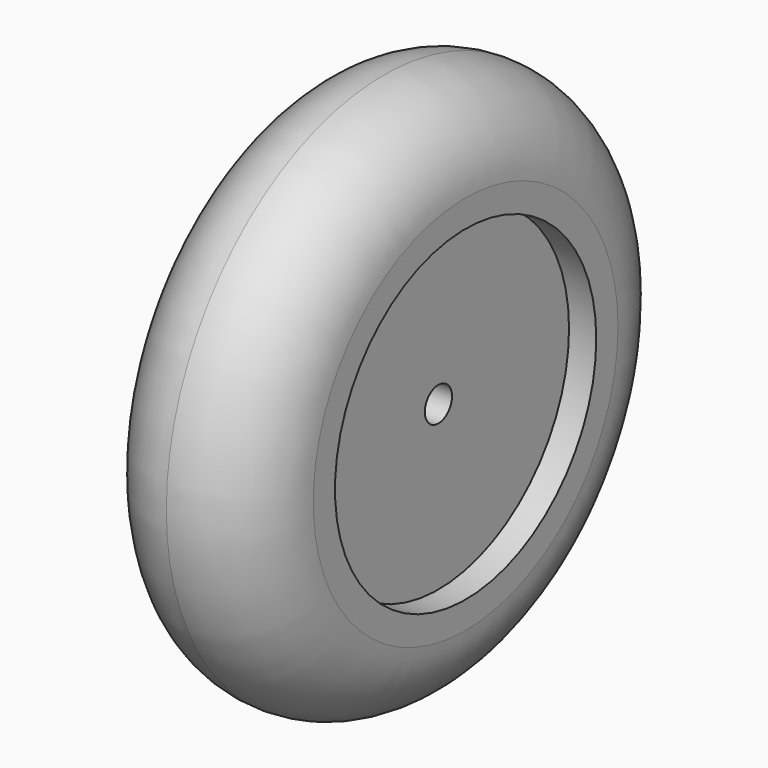
from build123d import *

# Parameters (mm, degrees)
F0_R     = 127
F0_R_2   = 76.2
F1_DEPTH = 38.1
F2_R     = 38.09999
F0_R_3   = 7.9375
F3_DEPTH = 25.4


# Not quite as in the source:
# - a fillet or chamfer is up to 0.001 mm smaller than in the source, because OpenCascade refuses the exact size


with BuildPart() as f1:
    # F0 (on Right) → F1 (new body, symmetric)
    with BuildSketch(Plane.YZ):
        Circle(F0_R)
        Circle(F0_R_2, mode=Mode.SUBTRACT)
    extrude(amount=F1_DEPTH, both=True)

    # F2 (radius 38.1 in the source; OpenCascade refuses exactly that, so slightly less here)
    f2_edges = [f1.edges().sort_by_distance(p)[0] for p in [
        (38.1, -127, 0),
        (-38.1, -127, 0),
    ]]
    fillet(f2_edges, radius=F2_R)

    # F0 (on Right) → F3 (join, symmetric)
    with BuildSketch(Plane.YZ):
        Circle(F0_R_2)
        Circle(F0_R_3, mode=Mode.SUBTRACT)
    extrude(amount=F3_DEPTH, both=True)


solid = f1.part
